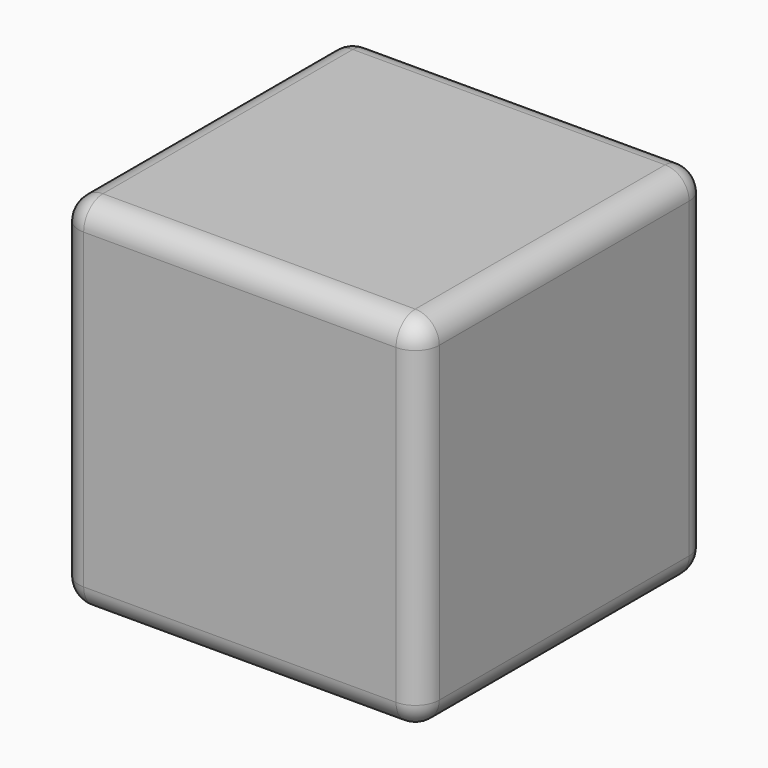
from build123d import *

# Parameters (mm, degrees)
F0_W     = 76.2
F0_H     = 76.2
F1_DEPTH = 76.2
F2_T     = -5.08
F3_R     = 5.07999


# Not quite as in the source:
# - a fillet or chamfer is up to 0.001 mm smaller than in the source, because OpenCascade refuses the exact size


with BuildPart() as f1:
    # F0 (on Front) → F1 (new body)
    with BuildSketch(Plane.XZ):
        with Locations((38.1, 38.1)):
            Rectangle(F0_W, F0_H)
    extrude(amount=F1_DEPTH)

    # F2
    f2_openings = [f1.faces().sort_by_distance(p)[0] for p in [
        (38.1, -38.1, 0),
    ]]
    offset(amount=F2_T, openings=f2_openings)

    # F3 (radius 5.08 in the source; OpenCascade refuses exactly that, so slightly less here)
    f3_edges = [f1.edges().sort_by_distance(p)[0] for p in [
        (76.2, -38.1, 76.2),
        (0, -38.1, 76.2),
        (38.1, 0, 76.2),
        (38.1, -76.2, 76.2),
        (76.2, -38.1, 0),
        (76.2, 0, 38.1),
        (76.2, -76.2, 38.1),
        (0, 0, 38.1),
        (0, -76.2, 38.1),
        (38.1, -76.2, 0),
        (0, -38.1, 0),
        (38.1, 0, 0),
    ]]
    fillet(f3_edges, radius=F3_R)


solid = f1.part
